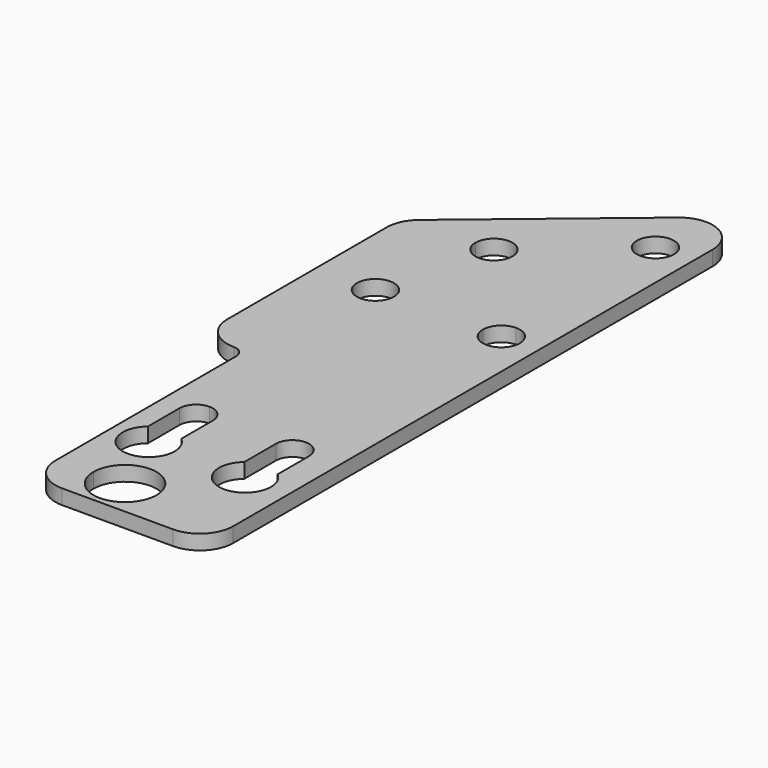
from build123d import *

# Parameters (mm, degrees)
F0_R     = 2.5
F1_DEPTH = 2
F2_R     = 4.5
F3_R     = 1.49999


# Not quite as in the source:
# - a fillet or chamfer is up to 0.001 mm smaller than in the source, because OpenCascade refuses the exact size


with BuildPart() as f1:
    # F0 (on Top) → F1 (new body)
    with BuildSketch(Plane.XY):
        with BuildLine():
            Line((6, -12.5), (12, -12.5))
            Line((12, -12.5), (12, 9.5))
            Line((12, 9.5), (8.25, 9.5))
            Line((8.25, 9.5), (8.25, 4.1809513237))
            ThreePointArc((8.25, 4.1809513237), (9.1721443851, 2.9790199458), (9.5, 1.5))
            ThreePointArc((9.5, 1.5), (8.4748737342, -0.9748737342), (6, -2))
            Line((6, -2), (6, -12.5))
        make_face()
        with BuildLine():
            Line((8.25, 9.5), (12, 9.5))
            Line((12, 9.5), (12, 12.5))
            Line((12, 12.5), (-7, 12.5))
            Line((-7, 12.5), (-7, 11.75))
            ThreePointArc((-7, 11.75), (-5.4090097423, 11.0909902577), (-4.75, 9.5))
            Line((-4.75, 9.5), (-4.75, 4.1809513237))
            ThreePointArc((-4.75, 4.1809513237), (-3.8278556149, 2.9790199458), (-3.5, 1.5))
            ThreePointArc((-3.5, 1.5), (-8.4790199458, -1.6721443851), (-9.25, 4.1809513237))
            Line((-9.25, 4.1809513237), (-9.25, 9.5))
            Line((-9.25, 9.5), (-12, 9.5))
            Line((-12, 9.5), (-12, -7.5))
            Line((-12, -7.5), (-7.25, -7.5))
            ThreePointArc((-7.25, -7.5), (-3, -3.25), (1.25, -7.5))
            ThreePointArc((1.25, -7.5), (0.00520382, -10.50520382), (-3, -11.75))
            Line((-3, -11.75), (-3, -12.5))
            Line((-3, -12.5), (6, -12.5))
            Line((6, -12.5), (6, -2))
            ThreePointArc((6, -2), (2.7111301612, 0.3027802276), (3.75, 4.1809513237))
            Line((3.75, 4.1809513237), (3.75, 9.5))
            ThreePointArc((3.75, 9.5), (6, 11.75), (8.25, 9.5))
        make_face()
        Polygon((-7, 12.5), (12, 12.5), (12, 22.5), (7, 22.5), (-6, 22.5), (-12, 22.5), (-12, 12.5), align=None)
        with BuildLine():
            Line((-12, -12.5), (-3, -12.5))
            Line((-3, -12.5), (-3, -11.75))
            ThreePointArc((-3, -11.75), (-6.00520382, -10.50520382), (-7.25, -7.5))
            Line((-7.25, -7.5), (-12, -7.5))
            Line((-12, -7.5), (-12, -12.5))
        make_face()
        with BuildLine():
            Line((-7, 11.75), (-7, 12.5))
            Line((-7, 12.5), (-12, 12.5))
            Line((-12, 12.5), (-12, 9.5))
            Line((-12, 9.5), (-9.25, 9.5))
            ThreePointArc((-9.25, 9.5), (-8.5909902577, 11.0909902577), (-7, 11.75))
        make_face()
        with BuildLine():
            Line((7, 22.5), (12, 22.5))
            Line((12, 22.5), (12, 43.5))
            Line((12, 43.5), (9.5, 43.5))
            ThreePointArc((9.5, 43.5), (8.767766953, 41.732233047), (7, 41))
            Line((7, 41), (7, 22.5))
        make_face()
        with BuildLine():
            Line((-6, 22.5), (7, 22.5))
            Line((7, 22.5), (7, 41))
            ThreePointArc((7, 41), (5.232233047, 41.732233047), (4.5, 43.5))
            Line((4.5, 43.5), (-6, 43.5))
            Line((-6, 43.5), (-6, 22.5))
        make_face()
        with BuildLine():
            Line((9.5, 43.5), (12, 43.5))
            Line((12, 43.5), (12, 72.5))
            Line((12, 72.5), (0, 72.5))
            Line((0, 72.5), (-16.8, 58.5))
            Line((-16.8, 58.5), (-8.5, 58.5))
            ThreePointArc((-8.5, 58.5), (-6, 61), (-3.5, 58.5))
            ThreePointArc((-3.5, 58.5), (-4.232233047, 56.732233047), (-6, 56))
            Line((-6, 56), (-6, 43.5))
            Line((-6, 43.5), (4.5, 43.5))
            ThreePointArc((4.5, 43.5), (5.232233047, 45.267766953), (7, 46))
            ThreePointArc((7, 46), (8.767766953, 45.267766953), (9.5, 43.5))
        make_face()
        with BuildLine():
            ThreePointArc((9.5, 69.5), (8.767766953, 67.732233047), (7, 67))
            ThreePointArc((7, 67), (5.232233047, 71.267766953), (9.5, 69.5))
        make_face(mode=Mode.SUBTRACT)
        with BuildLine():
            Line((-12, 24), (-12, 22.5))
            Line((-12, 22.5), (-6, 22.5))
            Line((-6, 22.5), (-6, 43.5))
            Line((-6, 43.5), (-6, 56))
            ThreePointArc((-6, 56), (-7.767766953, 56.732233047), (-8.5, 58.5))
            Line((-8.5, 58.5), (-16.8, 58.5))
            Line((-16.8, 58.5), (-18, 57.5))
            Line((-18, 57.5), (-18, 24))
            Line((-18, 24), (-12, 24))
        make_face()
        with Locations((-10, 43.5)):
            Circle(F0_R, mode=Mode.SUBTRACT)
        Polygon((0, 72.5), (12, 72.5), (12, 82.5), align=None)
    extrude(amount=F1_DEPTH)

    # F2
    f2_edges = [f1.edges().sort_by_distance(p)[0] for p in [
        (12, 82.5, 1),
        (-18, 57.5, 1),
        (-12, -12.5, 1),
        (12, -12.5, 1),
        (-18, 24, 1),
    ]]
    fillet(f2_edges, radius=F2_R)

    # F3 (radius 1.5 in the source; OpenCascade refuses exactly that, so slightly less here)
    f3_edges = [f1.edges().sort_by_distance(p)[0] for p in [
        (-12, 24, 1),
    ]]
    fillet(f3_edges, radius=F3_R)


solid = f1.part
